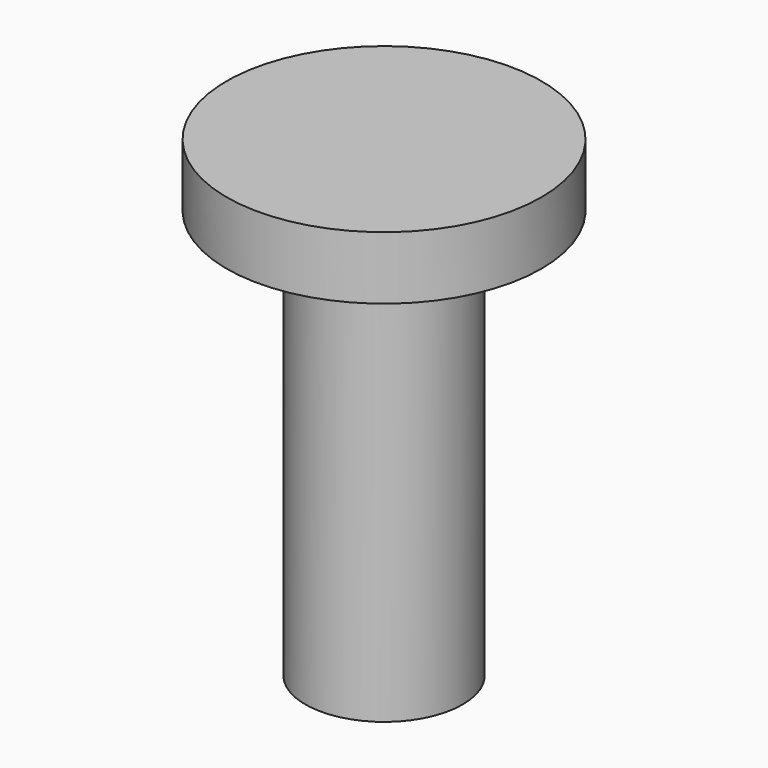
from build123d import *

# Parameters (mm, degrees)
F0_R     = 5
F2_DEPTH = 2
F3_R     = 2.5
F4_DEPTH = 13


# Not quite as in the source:
# - the program builds the solid bodies; features that only make, move or delete a surface that nothing else refers to are left out


with BuildPart() as f2:
    # F0 (on Top) → F2 (new body)
    with BuildSketch(Plane.XY):
        Circle(F0_R)
    extrude(amount=F2_DEPTH)

    # F3 (on Top) → F4 (join)
    with BuildSketch(Plane.XY):
        Circle(F3_R)
    extrude(amount=-F4_DEPTH)


solid = f2.part
